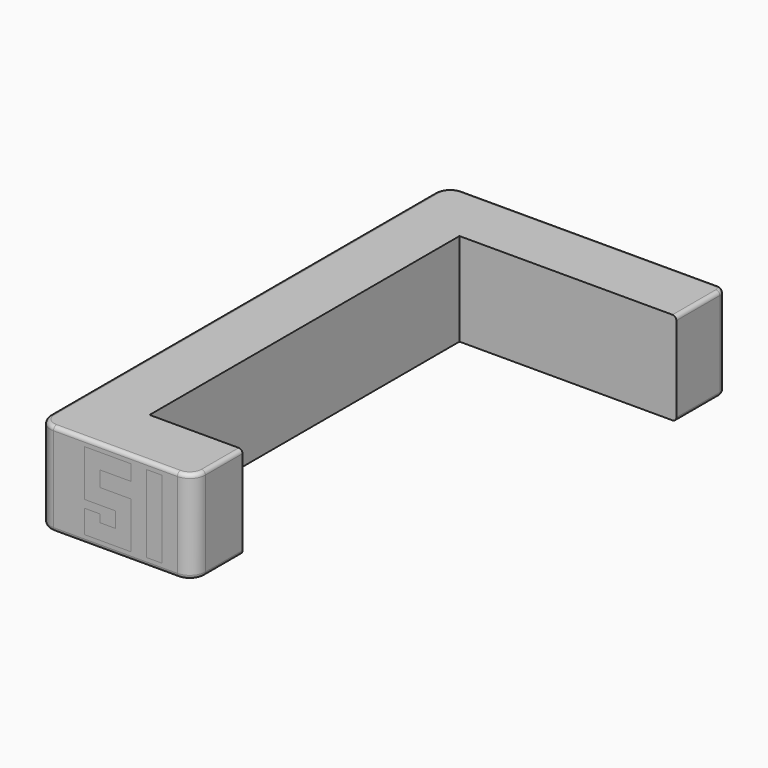
from build123d import *

# Parameters (mm, degrees)
F1_DEPTH  = 152.4
F2_R      = 25.4
F3_W      = 25.4
F3_H      = 127
F4_DEPTH  = 25.4
F5_DEPTH  = 25.4
F6_W      = 25.4
F6_H      = 127
F7_DEPTH  = 25.4
F8_DEPTH  = 25.4
F10_DEPTH = 25.4
F11_DEPTH = 25.4
F12_R     = 12.69999
F13_R     = 6.35


# Not quite as in the source:
# - a fillet or chamfer is up to 0.001 mm smaller than in the source, because OpenCascade refuses the exact size


with BuildPart() as f1:
    # F0 (on Top) → F1 (new body)
    with BuildSketch(Plane.XY):
        Polygon((355.6309728362, 708.7584971195), (-101.5690271638, 708.7584971195), (-101.5690271638, -129.4415028805), (152.4309728362, -129.4415028805), (152.4309728362, -27.8415028805), (0.0309728362, -27.8415028805), (0.0309728362, 607.1584971195), (355.6309728362, 607.1584971195), align=None)
    extrude(amount=F1_DEPTH)

    # F2
    f2_edges = [f1.edges().sort_by_distance(p)[0] for p in [
        (-101.569027, -129.441503, 76.2),
        (-101.569027, 708.758497, 76.2),
        (152.430973, -129.441503, 76.2),
    ]]
    fillet(f2_edges, radius=F2_R)

    # F3 (on face) → F4 (cut)
    with BuildSketch(Plane(origin=(-101.5690271638, 0, 0), x_dir=(0, -1, 0), z_dir=(-1, 0, 0))):
        Polygon((-384.9084971195, 114.3), (-384.9084971195, 139.7), (-461.1084971195, 139.7), (-461.1084971195, 63.5), (-410.3084971195, 63.5), (-410.3084971195, 38.1), (-435.7084971195, 38.1), (-435.7084971195, 50.8), (-461.1084971195, 50.8), (-461.1084971195, 12.7), (-384.9084971195, 12.7), (-384.9084971195, 88.9), (-435.7084971195, 88.9), (-435.7084971195, 114.3), align=None)
        with Locations((-346.8084971195, 76.2)):
            Rectangle(F3_W, F3_H)
        Polygon((-232.5084971195, 139.7), (-274.3105804205, 139.7), (-308.7084971195, 63.5), (-308.7084971195, 38.1), (-257.9084971195, 38.1), (-257.9084971195, 12.7), (-232.5084971195, 12.7), (-232.5084971195, 38.1), (-219.8084971195, 38.1), (-219.8084971195, 63.5), (-232.5084971195, 63.5), align=None)
        Polygon((-257.9084971195, 114.3), (-257.9084971195, 63.5), (-280.8404415855, 63.5), align=None, mode=Mode.SUBTRACT)
        Polygon((-118.2084971195, 114.3), (-118.2084971195, 139.7), (-194.4084971195, 139.7), (-194.4084971195, 63.5), (-143.6084971195, 63.5), (-143.6084971195, 38.1), (-169.0084971195, 38.1), (-169.0084971195, 50.8), (-194.4084971195, 50.8), (-194.4084971195, 12.7), (-118.2084971195, 12.7), (-118.2084971195, 88.9), (-169.0084971195, 88.9), (-169.0084971195, 114.3), align=None)
    extrude(amount=-F4_DEPTH, mode=Mode.SUBTRACT)


with BuildPart() as f5:
    # F5 (new): a face of the model
    f5_faces = [f1.part.faces().sort_by_distance(p)[0] for p in [
        (-76.1690271638, 424.1128449456, 74.8195652174),
    ]]
    extrude(f5_faces, amount=F5_DEPTH)


with BuildPart() as f5b:
    # F5#2 (new): a face of the model
    f5_2_faces = [f1.part.faces().sort_by_distance(p)[0] for p in [
        (-76.1690271638, 346.8084971195, 76.2),
    ]]
    extrude(f5_2_faces, amount=F5_DEPTH)


with BuildPart() as f5c:
    # F5#3 (new): a face of the model
    f5_3_faces = [f1.part.faces().sort_by_distance(p)[0] for p in [
        (-76.1690271638, 253.40953877, 138.1497674368),
    ]]
    extrude(f5_3_faces, amount=F5_DEPTH)


with BuildPart() as f5d:
    # F5#4 (new): a face of the model
    f5_4_faces = [f1.part.faces().sort_by_distance(p)[0] for p in [
        (-76.1690271638, 157.4128449456, 74.8195652174),
    ]]
    extrude(f5_4_faces, amount=F5_DEPTH)


with BuildPart() as f1_1:
    add(f1.part)

    # F6 (on face) → F7 (cut)
    with BuildSketch(Plane.XZ.offset(129.4415028805)):
        Polygon((50.8309728362, 114.3), (50.8309728362, 139.7), (-25.3690271638, 139.7), (-25.3690271638, 63.5), (25.4309728362, 63.5), (25.4309728362, 38.1), (0.0309728362, 38.1), (0.0309728362, 50.8), (-25.3690271638, 50.8), (-25.3690271638, 12.7), (50.8309728362, 12.7), (50.8309728362, 88.9), (0.0309728362, 88.9), (0.0309728362, 114.3), align=None)
        with Locations((88.9309728362, 76.2)):
            Rectangle(F6_W, F6_H)
    extrude(amount=-F7_DEPTH, mode=Mode.SUBTRACT)


with BuildPart() as f8:
    # F8 (new): a face of the model
    f8_faces = [f1_1.part.faces().sort_by_distance(p)[0] for p in [
        (11.6266250101, -104.0415028805, 74.8195652174),
    ]]
    extrude(f8_faces, amount=F8_DEPTH)


with BuildPart() as f8b:
    # F8#2 (new): a face of the model
    f8_2_faces = [f1_1.part.faces().sort_by_distance(p)[0] for p in [
        (88.9309728362, -104.0415028805, 76.2),
    ]]
    extrude(f8_2_faces, amount=F8_DEPTH)


with BuildPart() as f1_2:
    add(f1_1.part)

    # F9 (on face) → F10 (cut)
    with BuildSketch(Plane(origin=(0, 708.7584971195, 0), x_dir=(-1, 0, 0), z_dir=(0, 1, 0))):
        Polygon((-266.7309728362, 139.7), (-308.5330561372, 139.7), (-342.9309728362, 63.5), (-342.9309728362, 38.1), (-292.1309728362, 38.1), (-292.1309728362, 12.7), (-266.7309728362, 12.7), (-266.7309728362, 38.1), (-254.0309728362, 38.1), (-254.0309728362, 63.5), (-266.7309728362, 63.5), align=None)
        Polygon((-292.1309728362, 63.5), (-315.0629173021, 63.5), (-292.1309728362, 114.3), align=None, mode=Mode.SUBTRACT)
        Polygon((-152.4309728362, 114.3), (-152.4309728362, 139.7), (-228.6309728362, 139.7), (-228.6309728362, 63.5), (-177.8309728362, 63.5), (-177.8309728362, 38.1), (-203.2309728362, 38.1), (-203.2309728362, 50.8), (-228.6309728362, 50.8), (-228.6309728362, 12.7), (-152.4309728362, 12.7), (-152.4309728362, 88.9), (-203.2309728362, 88.9), (-203.2309728362, 114.3), align=None)
    extrude(amount=-F10_DEPTH, mode=Mode.SUBTRACT)


with BuildPart() as f11:
    # F11 (new): a face of the model
    f11_faces = [f1_2.part.faces().sort_by_distance(p)[0] for p in [
        (287.6320144867, 683.3584971195, 138.1497674368),
    ]]
    extrude(f11_faces, amount=F11_DEPTH)


with BuildPart() as f11b:
    # F11#2 (new): a face of the model
    f11_2_faces = [f1_2.part.faces().sort_by_distance(p)[0] for p in [
        (191.6353206623, 683.3584971195, 74.8195652174),
    ]]
    extrude(f11_2_faces, amount=F11_DEPTH)


with BuildPart() as f1_3:
    add(f1_2.part)

    # F12 (radius 12.7 in the source; OpenCascade refuses exactly that, so slightly less here)
    f12_edges = [f1_3.edges().sort_by_distance(p)[0] for p in [
        (355.630973, 708.758497, 76.2),
    ]]
    fillet(f12_edges, radius=F12_R)

    # F13
    f13_edges = [f1_3.edges().sort_by_distance(p)[0] for p in [
        (25.430973, -129.441503, 152.4),
        (25.430973, -129.441503, 0),
    ]]
    fillet(f13_edges, radius=F13_R)


solid = Compound([f5.part, f5b.part, f5c.part, f5d.part, f8.part, f8b.part, f11.part, f11b.part, f1_3.part])
